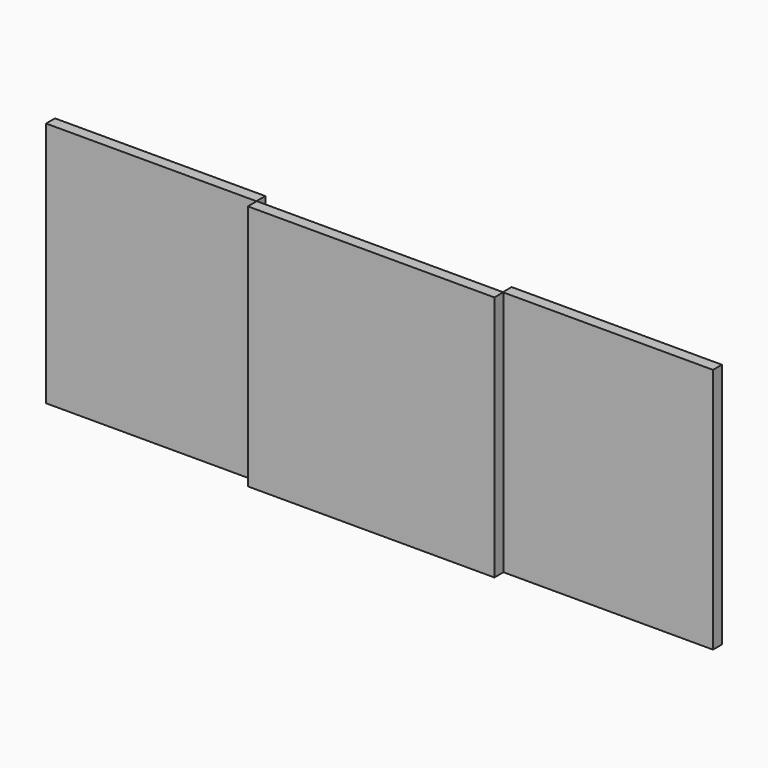
from build123d import *

# Parameters (mm, degrees)
F0_W     = 82.199988
F0_H     = 82.199988
F2_DEPTH = 3.719999926
F1_W     = 70.1101869345
F1_H     = 82.1198001504
F3_DEPTH = 3.719999926


# Not quite as in the source:
# - a feature of the source that left no trace in its solid (it failed there, or was rolled back) is left out


with BuildPart() as f2:
    # F0 (on Front) → F2 (new body)
    with BuildSketch(Plane.XZ):
        Rectangle(F0_W, F0_H)
    extrude(amount=F2_DEPTH)

    # F1 (on Front) → F3, piece 2 (join)
    with BuildSketch(Plane.XZ):
        with Locations((75.9527012706, 0)):
            Rectangle(F1_W, F1_H)
    extrude(amount=-F3_DEPTH)


with BuildPart() as f3:
    # F1 (on Front) → F3 (new body)
    with BuildSketch(Plane.XZ):
        with Locations((-76.2772858143, 0)):
            Rectangle(F1_W, F1_H)
    extrude(amount=-F3_DEPTH)


solid = Compound([f2.part, f3.part])
